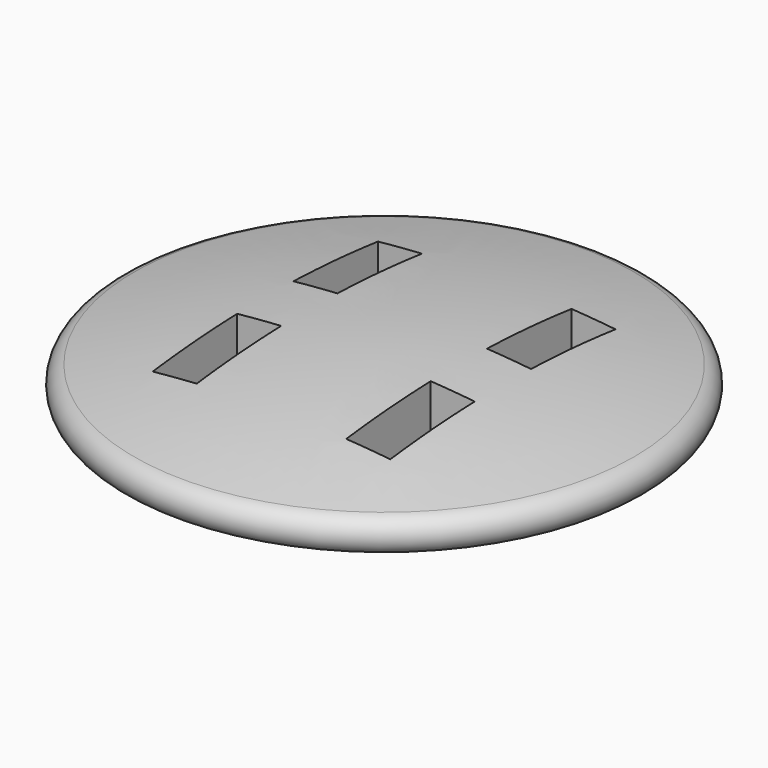
from build123d import *

# Parameters (mm, degrees)
F2_W             = 50
F2_H             = 120
F3_DEPTH         = 50.001
F3_DEPTH_BACK    = 50.001
F3_COPIES2_COUNT = 2


# Not quite as in the source:
# - a pattern or mirror of a feature is missing from the dataset's text; its kind, count and spacing are read off the source's solid


with BuildPart() as f1:
    # F0 (on Front) → F1 (revolve)
    with BuildSketch(Plane.XZ):
        with BuildLine():
            ThreePointArc((284.237074401, -19.5460277427), (300, 0), (284.237074401, 19.5460277427))
            ThreePointArc((284.237074401, 19.5460277427), (142.931940876, 42.3647815091), (0, 50))
            Line((0, 50), (0, -50))
            ThreePointArc((0, -50), (142.931940876, -42.3647815091), (284.237074401, -19.5460277428))
        make_face()
    revolve(axis=Axis((0, 0, 0), (0, 0, -1)))

    # F2 (on Top) → F3 (cut, two sides)
    with BuildSketch(Plane.XY) as f3_sk:
        with Locations((-110, 100)):
            Rectangle(F2_W, F2_H)
    f3 = extrude(amount=-F3_DEPTH, mode=Mode.SUBTRACT) + extrude(f3_sk.sketch, amount=F3_DEPTH_BACK, mode=Mode.SUBTRACT)

    # F3_copies: F3 across plane
    add(f3.mirror(Plane(origin=(0, 0, 0), x_dir=(0, 0, 1), z_dir=(1, 0, 0))), mode=Mode.SUBTRACT)

    # F3_copies1: F3 across plane
    add(f3.mirror(Plane(origin=(0, 0, 0), x_dir=(0, 0, -1), z_dir=(0, -1, 0))), mode=Mode.SUBTRACT)

    # F3_copies2: F3 ×2 about axis
    f3_copies2_axis = Axis((0, 0, 0), (0, 0, 1))
    for i in range(1, F3_COPIES2_COUNT):
        add(f3.rotate(f3_copies2_axis, i * 360 / F3_COPIES2_COUNT), mode=Mode.SUBTRACT)


solid = f1.part
